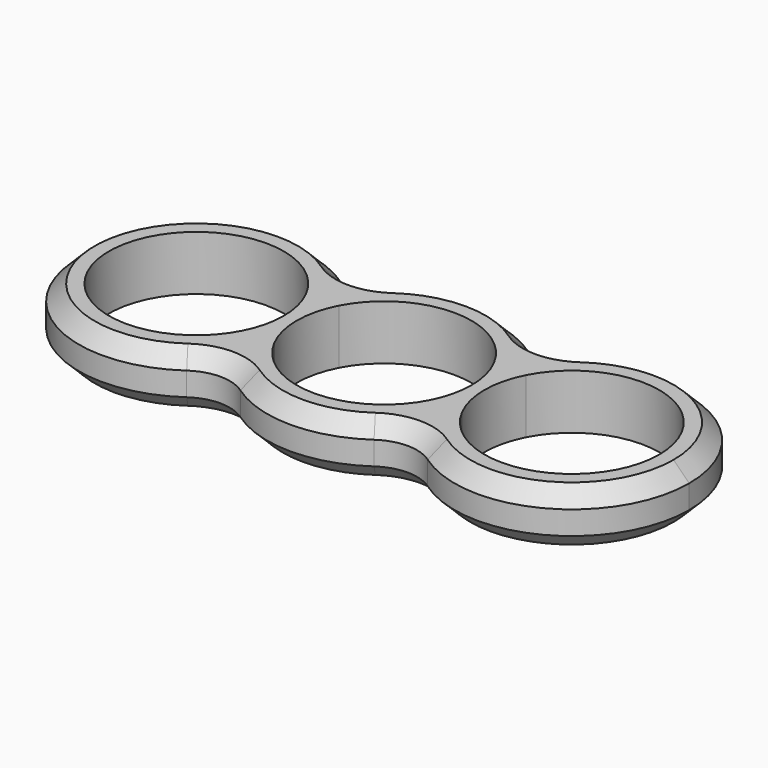
from build123d import *

# Parameters (mm, degrees)
F1_DEPTH = 7
F2_R     = 6
F3_SIZE  = 2


# Not quite as in the source:
# - a feature names something its author has since deleted; it is built from what else it names


with BuildPart() as f1:
    # F0 (on Top) → F1 (new body)
    with BuildSketch(Plane.XY):
        with BuildLine():
            ThreePointArc((-14.0623969756, 5.1112299037), (-13.1615738007, 7.1167868393), (-11.9765766631, 8.9686839202))
            ThreePointArc((-11.9765766631, 8.9686839202), (-39, 0), (-11.9765766631, -8.9686839202))
            ThreePointArc((-11.9765766631, -8.9686839202), (-13.1615738007, -7.1167868393), (-14.0623969756, -5.1112299037))
            ThreePointArc((-14.0623969756, -5.1112299037), (-35.175, 0), (-14.0623969756, 5.1112299037))
        make_face()
        with BuildLine():
            ThreePointArc((-9.9141796875, -5.1565168597), (-11.175, 0), (-9.9141796875, 5.1565168597))
            ThreePointArc((-9.9141796875, 5.1565168597), (-10.8069599633, 7.1374851726), (-11.9765766631, 8.9686839202))
            ThreePointArc((-11.9765766631, 8.9686839202), (-13.1615738007, 7.1167868393), (-14.0623969756, 5.1112299037))
            ThreePointArc((-14.0623969756, 5.1112299037), (-13.1387537824, 2.6294401687), (-12.825, 0))
            ThreePointArc((-12.825, 0), (-13.1387537824, -2.6294401687), (-14.0623969756, -5.1112299037))
            ThreePointArc((-14.0623969756, -5.1112299037), (-13.1615738007, -7.1167868393), (-11.9765766631, -8.9686839202))
            ThreePointArc((-11.9765766631, -8.9686839202), (-10.8069599633, -7.1374851726), (-9.9141796875, -5.1565168597))
        make_face()
        with BuildLine():
            ThreePointArc((-9.9141796875, 5.1565168597), (0, 11.175), (9.9141796875, 5.1565168597))
            ThreePointArc((9.9141796875, 5.1565168597), (10.8069599633, 7.1374851726), (11.9765766631, 8.9686839202))
            ThreePointArc((11.9765766631, 8.9686839202), (0, 14.9624757252), (-11.9765766631, 8.9686839202))
            ThreePointArc((-11.9765766631, 8.9686839202), (-10.8069599633, 7.1374851726), (-9.9141796875, 5.1565168597))
        make_face()
        with BuildLine():
            ThreePointArc((9.9141796875, 5.1565168597), (10.8552195512, 2.6542105222), (11.175, 0))
            ThreePointArc((11.175, 0), (10.8552195512, -2.6542105222), (9.9141796875, -5.1565168597))
            ThreePointArc((9.9141796875, -5.1565168597), (10.8069599633, -7.1374851726), (11.9765766631, -8.9686839202))
            ThreePointArc((11.9765766631, -8.9686839202), (13.1615738007, -7.1167868393), (14.0623969756, -5.1112299037))
            ThreePointArc((14.0623969756, -5.1112299037), (12.825, 0), (14.0623969756, 5.1112299037))
            ThreePointArc((14.0623969756, 5.1112299037), (13.1615738007, 7.1167868393), (11.9765766631, 8.9686839202))
            ThreePointArc((11.9765766631, 8.9686839202), (10.8069599633, 7.1374851726), (9.9141796875, 5.1565168597))
        make_face()
        with BuildLine():
            ThreePointArc((39, 0), (28.724862429, 14.2364207239), (11.9765766631, 8.9686839202))
            ThreePointArc((11.9765766631, 8.9686839202), (13.1615738007, 7.1167868393), (14.0623969756, 5.1112299037))
            ThreePointArc((14.0623969756, 5.1112299037), (26.6294401687, 10.8612462176), (35.175, 0))
            ThreePointArc((35.175, 0), (26.6294401687, -10.8612462176), (14.0623969756, -5.1112299037))
            ThreePointArc((14.0623969756, -5.1112299037), (13.1615738007, -7.1167868393), (11.9765766631, -8.9686839202))
            ThreePointArc((11.9765766631, -8.9686839202), (28.724862429, -14.2364207239), (39, 0))
        make_face()
        with BuildLine():
            ThreePointArc((11.9765766631, -8.9686839202), (10.8069599633, -7.1374851726), (9.9141796875, -5.1565168597))
            ThreePointArc((9.9141796875, -5.1565168597), (0, -11.175), (-9.9141796875, -5.1565168597))
            ThreePointArc((-9.9141796875, -5.1565168597), (-10.8069599633, -7.1374851726), (-11.9765766631, -8.9686839202))
            ThreePointArc((-11.9765766631, -8.9686839202), (0, -14.9624757252), (11.9765766631, -8.9686839202))
        make_face()
    extrude(amount=F1_DEPTH)

    # F2
    f2_edges = [f1.edges().sort_by_distance(p)[0] for p in [
        (-11.976577, -8.968684, 3.5),
        (11.976577, -8.968684, 3.5),
        (11.976577, 8.968684, 3.5),
        (-11.976577, 8.968684, 3.5),
    ]]
    fillet(f2_edges, radius=F2_R)

    # F3
    f3_edges = [f1.edges().sort_by_distance(p)[0] for p in [
        (-39, 0, 0),
        (-39, 0, 7),
    ]]
    chamfer(f3_edges, length=F3_SIZE)


solid = f1.part
